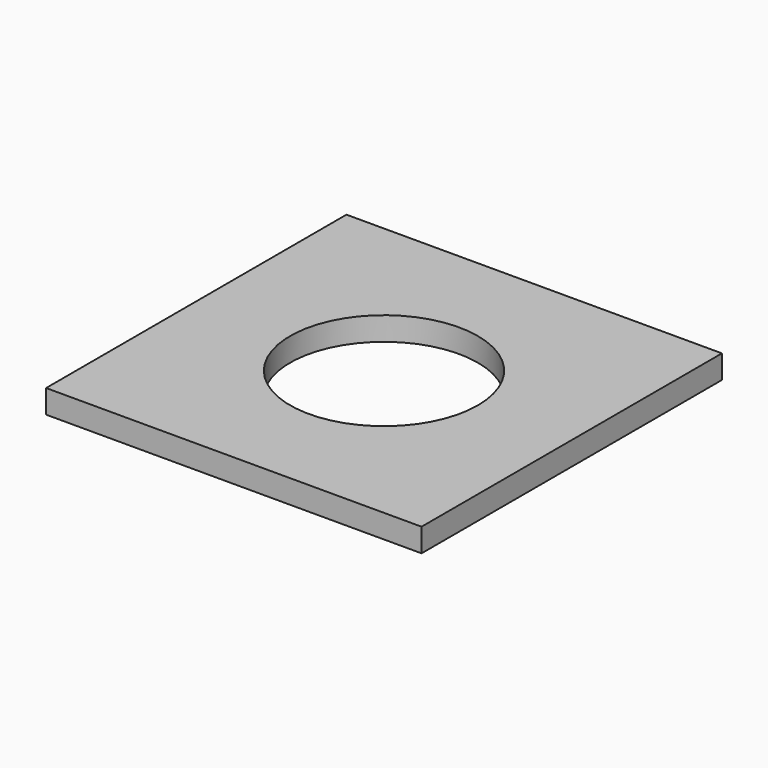
from build123d import *

# Parameters (mm, degrees)
F0_W     = 50.8
F0_H     = 50.8
F0_R     = 12.7
F1_DEPTH = 3.175


# Not quite as in the source:
# - a length typed as a fraction of an inch, garbled in the dataset ("3 / 203.2 mm" for 3/8 in), is restored


with BuildPart() as f1:
    # F0 (on Top) → F1 (new body)
    with BuildSketch(Plane.XY):
        with Locations((-25.4, 0)):
            Rectangle(F0_W, F0_H)
        with Locations((-25.4, 0)):
            Circle(F0_R, mode=Mode.SUBTRACT)
    extrude(amount=F1_DEPTH)


solid = f1.part
